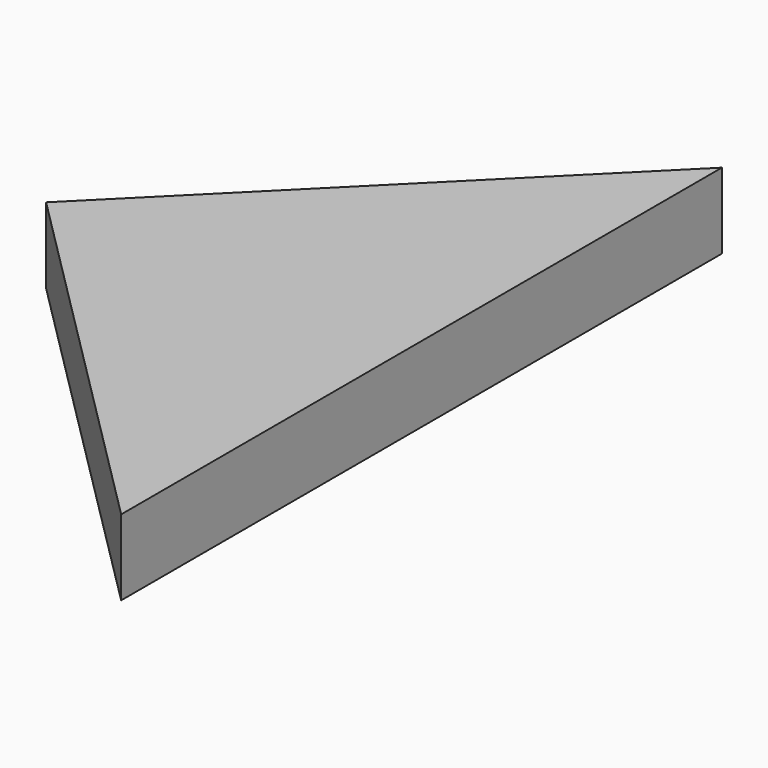
from build123d import *

# Parameters (mm, degrees)
F3_DEPTH = 4.826


# Not quite as in the source:
# - the program builds the solid bodies; features that only make, move or delete a surface that nothing else refers to are left out


with BuildPart() as f3:
    # F2 (on Top) → F3 (new body, symmetric)
    with BuildSketch(Plane.XY):
        Polygon((24.3828949223, 47.8737466673), (-23.490851745, 0), (24.3828949223, -47.8737466673), align=None)
    extrude(amount=F3_DEPTH, both=True)


solid = f3.part
